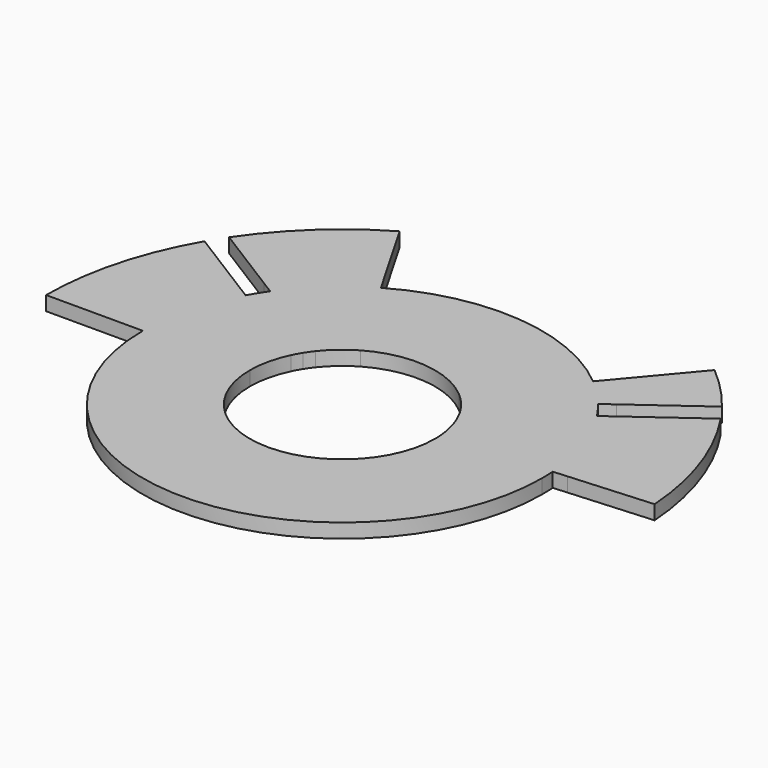
from build123d import *

# Parameters (mm, degrees)
F1_DEPTH = 1.4


# Not quite as in the source:
# - a feature names something its author has since deleted; it is built from what else it names


with BuildPart() as f1:
    # F0 (on Top) → F1 (new body)
    with BuildSketch(Plane.XY):
        with BuildLine():
            Line((9.1, 0), (19.6, 0))
            ThreePointArc((19.6, 0), (19.5880602096, 0.6840301354), (19.5522553851, 1.3672268854))
            Line((19.5522553851, 1.3672268854), (9.0778328574, 0.6347839111))
            ThreePointArc((9.0778328574, 0.6347839111), (9.0944565259, 0.31758542), (9.1, 0))
        make_face()
        with BuildLine():
            ThreePointArc((-19.6, 0), (0, -19.6), (19.6, 0))
            Line((19.6, 0), (9.1, 0))
            ThreePointArc((9.1, 0), (0, -9.1), (-9.1, 0))
            Line((-9.1, 0), (-19.6, 0))
        make_face()
        with BuildLine():
            Line((9.0778328574, 0.6347839111), (19.5522553851, 1.3672268854))
            ThreePointArc((19.5522553851, 1.3672268854), (18.5830433274, 6.2314124156), (16.4238667052, 10.6965696581))
            Line((16.4238667052, 10.6965696581), (7.9052534042, 4.5074348153))
            ThreePointArc((7.9052534042, 4.5074348153), (8.7095155433, 2.6371080753), (9.0778328574, 0.6347839111))
        make_face()
        with BuildLine():
            ThreePointArc((16.4238667052, 10.6965696581), (18.5830433274, 6.2314124156), (19.5522553851, 1.3672268854))
            Line((19.5522553851, 1.3672268854), (20.9488450555, 1.4648859486))
            ThreePointArc((20.9488450555, 1.4648859486), (19.8990062518, 6.7104061122), (17.5578688927, 11.5204704742))
            Line((17.5578688927, 11.5204704742), (16.4238667052, 10.6965696581))
        make_face()
        with BuildLine():
            Line((-21, 0), (-19.6, 0))
            ThreePointArc((-19.6, 0), (-18.9724573243, 4.9199454342), (-17.1300139719, 9.5248423254))
            Line((-17.1300139719, 9.5248423254), (-18.3187262027, 10.2676321667))
            ThreePointArc((-18.3187262027, 10.2676321667), (-20.3186275405, 5.3059753931), (-21, 0))
        make_face()
        with BuildLine():
            ThreePointArc((-17.1300139719, 9.5248423254), (-18.9724573243, 4.9199454342), (-19.6, 0))
            Line((-19.6, 0), (-9.1, 0))
            ThreePointArc((-9.1, 0), (-8.8722549614, 2.0231391203), (-8.2004193626, 3.9450123291))
            Line((-8.2004193626, 3.9450123291), (-17.1300139719, 9.5248423254))
        make_face()
        with BuildLine():
            Line((7.9052534042, 4.5074348153), (16.4238667052, 10.6965696581))
            ThreePointArc((16.4238667052, 10.6965696581), (16.1455577033, 11.1121989925), (15.8567330897, 11.5205909449))
            Line((15.8567330897, 11.5205909449), (7.3620546488, 5.3488457959))
            ThreePointArc((7.3620546488, 5.3488457959), (7.6452381851, 4.9356188157), (7.9052534042, 4.5074348153))
        make_face()
        with BuildLine():
            ThreePointArc((17.5578688927, 11.5204704742), (19.8990062518, 6.7104061122), (20.9488450555, 1.4648859486))
            Line((20.9488450555, 1.4648859486), (29.0291138626, 2.029913386))
            ThreePointArc((29.0291138626, 2.029913386), (27.512052622, 9.481400768), (24.1162750467, 16.285431461))
            Line((24.1162750467, 16.285431461), (17.5578688927, 11.5204704742))
        make_face()
        with BuildLine():
            ThreePointArc((-16.6217426847, 10.386417579), (-16.8813757535, 9.9588730623), (-17.1300139719, 9.5248423254))
            Line((-17.1300139719, 9.5248423254), (-8.2004193626, 3.9450123291))
            ThreePointArc((-8.2004193626, 3.9450123291), (-7.9709061334, 4.3902910396), (-7.717237675, 4.8222653045))
            Line((-7.717237675, 4.8222653045), (-16.6217426847, 10.386417579))
        make_face()
        with BuildLine():
            Line((-29.1, 0), (-21, 0))
            ThreePointArc((-21, 0), (-20.3186275405, 5.3059753931), (-18.3187262027, 10.2676321667))
            Line((-18.3187262027, 10.2676321667), (-25.1935432849, 14.5634946614))
            ThreePointArc((-25.1935432849, 14.5634946614), (-28.1064237283, 7.5391607759), (-29.1, 0))
        make_face()
        with BuildLine():
            Line((7.3620546488, 5.3488457959), (15.8567330897, 11.5205909449))
            ThreePointArc((15.8567330897, 11.5205909449), (15.5575809762, 11.9214795294), (15.2482962006, 12.3146036469))
            Line((15.2482962006, 12.3146036469), (6.7296828997, 6.1254688041))
            ThreePointArc((6.7296828997, 6.1254688041), (7.0565609618, 5.7458635027), (7.3620546488, 5.3488457959))
        make_face()
        with BuildLine():
            ThreePointArc((-16.0701754434, 11.2209385177), (-16.3512838646, 10.8071974155), (-16.6217426847, 10.386417579))
            Line((-16.6217426847, 10.386417579), (-7.717237675, 4.8222653045))
            ThreePointArc((-7.717237675, 4.8222653045), (-7.4401827106, 5.2396260586), (-7.1405808342, 5.6411085215))
            Line((-7.1405808342, 5.6411085215), (-16.0701754434, 11.2209385177))
        make_face()
        with BuildLine():
            Line((6.7296828997, 6.1254688041), (15.2482962006, 12.3146036469))
            ThreePointArc((15.2482962006, 12.3146036469), (13.9887542441, 13.7286108073), (12.5986371499, 15.0144710851))
            Line((12.5986371499, 15.0144710851), (5.8493672481, 6.9710044324))
            ThreePointArc((5.8493672481, 6.9710044324), (6.3037178141, 6.5630131586), (6.7296828997, 6.1254688041))
        make_face()
        with BuildLine():
            ThreePointArc((12.5986371499, 15.0144710851), (13.9887542441, 13.7286108073), (15.2482962006, 12.3146036469))
            Line((15.2482962006, 12.3146036469), (16.3822983881, 13.1385044629))
            ThreePointArc((16.3822983881, 13.1385044629), (15.0129754185, 14.6836837709), (13.4985398034, 16.0869333055))
            Line((13.4985398034, 16.0869333055), (12.5986371499, 15.0144710851))
        make_face()
        with BuildLine():
            Line((-17.2588876742, 11.963728359), (-16.0701754434, 11.2209385177))
            ThreePointArc((-16.0701754434, 11.2209385177), (-13.2510831681, 14.4419110533), (-9.8, 16.9740979142))
            Line((-9.8, 16.9740979142), (-10.5, 18.1865334795))
            ThreePointArc((-10.5, 18.1865334795), (-14.2239160262, 15.4492787172), (-17.2588876742, 11.963728359))
        make_face()
        with BuildLine():
            ThreePointArc((-9.8, 16.9740979142), (-13.2510831681, 14.4419110533), (-16.0701754434, 11.2209385177))
            Line((-16.0701754434, 11.2209385177), (-7.1405808342, 5.6411085215))
            ThreePointArc((-7.1405808342, 5.6411085215), (-5.9515972184, 6.8839298769), (-4.55, 7.8808311744))
            Line((-4.55, 7.8808311744), (-9.8, 16.9740979142))
        make_face()
        with BuildLine():
            Line((5.8493672481, 6.9710044324), (12.5986371499, 15.0144710851))
            ThreePointArc((12.5986371499, 15.0144710851), (1.7082525579, 19.5254160826), (-9.8, 16.9740979142))
            Line((-9.8, 16.9740979142), (-4.55, 7.8808311744))
            ThreePointArc((-4.55, 7.8808311744), (0.793117259, 9.0653717526), (5.8493672481, 6.9710044324))
        make_face()
        with BuildLine():
            ThreePointArc((13.4985398034, 16.0869333055), (15.0129754185, 14.6836837709), (16.3822983881, 13.1385044629))
            Line((16.3822983881, 13.1385044629), (22.9407045421, 17.9034654498))
            ThreePointArc((22.9407045421, 17.9034654498), (20.9382004615, 20.2089525071), (18.7051194419, 22.2918932948))
            Line((18.7051194419, 22.2918932948), (13.4985398034, 16.0869333055))
        make_face()
        with BuildLine():
            Line((-24.1337047564, 16.2595908537), (-17.2588876742, 11.963728359))
            ThreePointArc((-17.2588876742, 11.963728359), (-14.2239160262, 15.4492787172), (-10.5, 18.1865334795))
            Line((-10.5, 18.1865334795), (-14.55, 25.2013392501))
            ThreePointArc((-14.55, 25.2013392501), (-19.8518505313, 21.2770775832), (-24.1337047564, 16.2595908537))
        make_face()
    extrude(amount=F1_DEPTH)


solid = f1.part
